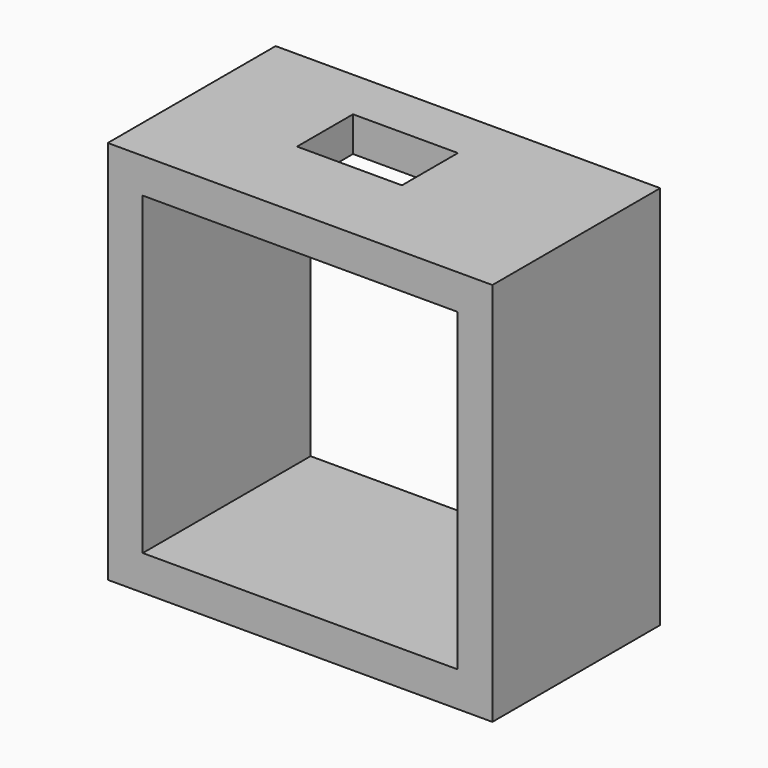
from build123d import *

# Parameters (mm, degrees)
F0_W     = 55
F0_H     = 55
F0_W_2   = 45
F0_H_2   = 45
F1_DEPTH = 30
F2_W     = 15
F2_H     = 10
F3_DEPTH = 25


# Not quite as in the source:
# - a feature names something its author has since deleted; it is built from what else it names


with BuildPart() as f1:
    # F0 (on Front) → F1 (new body)
    with BuildSketch(Plane.XZ):
        Rectangle(F0_W, F0_H)
        Rectangle(F0_W_2, F0_H_2, mode=Mode.SUBTRACT)
    extrude(amount=F1_DEPTH)

    # F2 (on face) → F3 (cut)
    with BuildSketch(Plane.XY.offset(27.5)):
        with Locations((-2.9486052878, -12.4806062132)):
            Rectangle(F2_W, F2_H)
    extrude(amount=-F3_DEPTH, mode=Mode.SUBTRACT)


solid = f1.part
